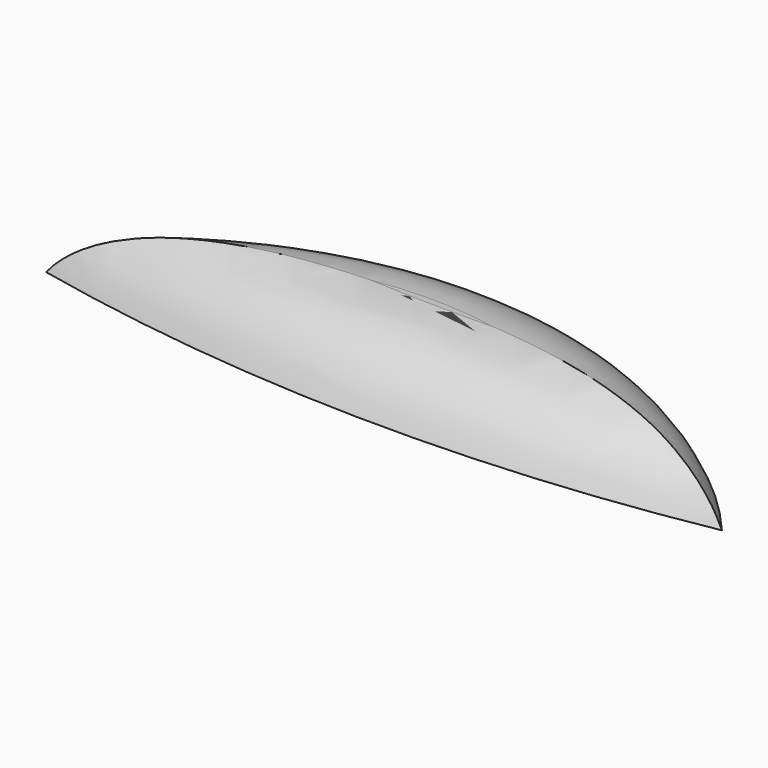
from build123d import *

# Parameters (mm, degrees)
F1_DEPTH    = 100
F2_T2_ANGLE = 37.7488316787
F2_T4_ANGLE = 155.3558475239


# Not quite as in the source:
# - a fillet or chamfer that OpenCascade refuses, or shapes differently, is made with other operations: its cross-section is extruded or revolved along the edge and cut away or added


with BuildPart() as f1:
    # F0 (on Top) → F1 (new body)
    with BuildSketch(Plane.XY):
        with BuildLine():
            ThreePointArc((-540.4781699181, -239.4952774048), (5.5714483543, -302.8761576492), (553.4174442291, -257.5761973858))
            ThreePointArc((553.4174442291, -257.5761973858), (10.5760494997, -0.097800723), (-540.4781699181, -239.4952774048))
        make_face()
    extrude(amount=F1_DEPTH)

    # F2: fillet of radius 156.7 on 2 edges, made by hand

    # F2_s1 → F2_t2 (revolve, cut)
    with BuildSketch(Plane(origin=(-744.5245583311, 268.3590209284, 0), x_dir=(0, 0, 1), z_dir=(-0.9407543779, 0.3390887795, 0))):
        with BuildLine():
            ThreePointArc((0, -432.5303133462), (72.6054136531, -374.9636800472), (100, -286.4481446876))
            Line((100, -286.4481446876), (100, -432.5303133462))
            Line((100, -432.5303133462), (0, -432.5303133462))
        make_face()
    revolve(axis=Axis((51.517612373, 2476.8666518852, 100), (0, 0, 1)), revolution_arc=F2_T2_ANGLE, mode=Mode.SUBTRACT)

    # F2_s3 → F2_t4 (revolve, cut)
    with BuildSketch(Plane(origin=(140.3959083331, -697.8496584538, 0), x_dir=(0, 0, 1), z_dir=(0.1972317322, -0.9803568961, 0))):
        with BuildLine():
            ThreePointArc((0, -581.717581759), (72.6054136531, -524.15094846), (100, -435.6354131004))
            Line((100, -435.6354131004), (100, -581.717581759))
            Line((100, -581.717581759), (0, -581.717581759))
        make_face()
    revolve(axis=Axis((-1.4286556925, -726.382435176, 100), (0, 0, 1)), revolution_arc=F2_T4_ANGLE, mode=Mode.SUBTRACT)


solid = f1.part
